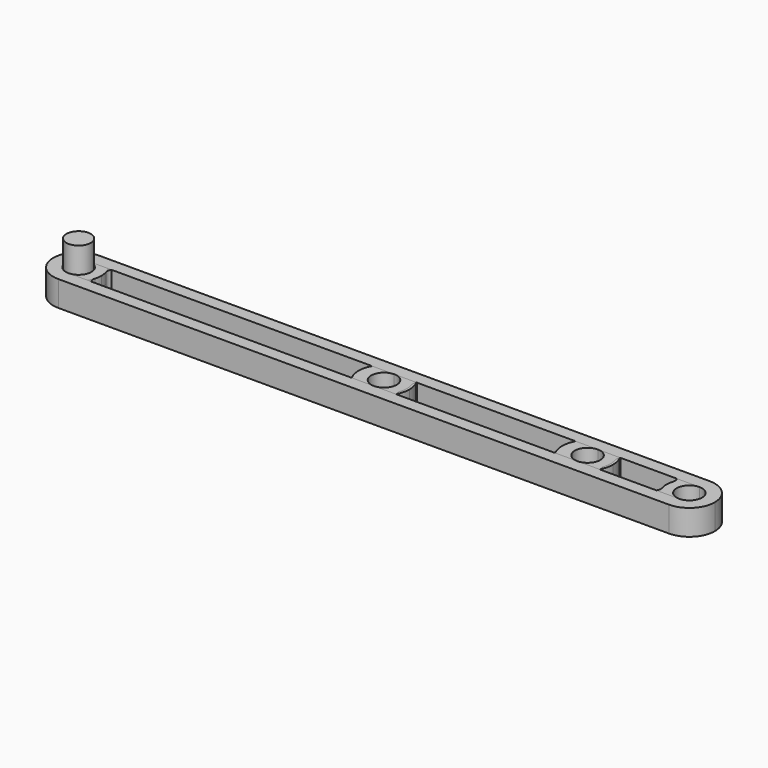
from build123d import *

# Parameters (mm, degrees)
F1_DEPTH      = 6.35
F2_DEPTH      = 6.35
F3_DEPTH      = 6.35
F4_DEPTH      = 6.35
F0_R          = 3.048
F5_DEPTH      = 12.7
F6_T          = -2.54
F7_T          = -2.54
F8_T          = -2.54
F9_T1_DEPTH   = 6.35
F9_2_T1_DEPTH = 6.35
F9_3_T1_DEPTH = 6.35


# Not quite as in the source:
# - a fillet or chamfer that OpenCascade refuses, or shapes differently, is made with other operations: its cross-section is extruded or revolved along the edge and cut away or added
# - two fillets or chamfers of one size are made in one step


with BuildPart() as f1:
    # F0 (on Top) → F1 (new body)
    with BuildSketch(Plane.XY):
        with BuildLine():
            ThreePointArc((0, 6.35), (3.175, 5.499261314), (5.499261314, 3.175))
            Line((5.499261314, 3.175), (70.700738686, 3.175))
            ThreePointArc((70.700738686, 3.175), (73.025, 5.499261314), (76.2, 6.35))
            Line((76.2, 6.35), (0, 6.35))
        make_face()
        with BuildLine():
            Line((76.2, 3.175), (70.700738686, 3.175))
            ThreePointArc((70.700738686, 3.175), (69.85, 0), (70.700738686, -3.175))
            Line((70.700738686, -3.175), (76.2, -3.175))
            ThreePointArc((76.2, -3.175), (73.025, 0), (76.2, 3.175))
        make_face()
        with BuildLine():
            Line((81.699261314, 3.175), (76.2, 3.175))
            ThreePointArc((76.2, 3.175), (78.4450640303, 2.2450640303), (79.375, 0))
            ThreePointArc((79.375, 0), (78.4450640303, -2.2450640303), (76.2, -3.175))
            Line((76.2, -3.175), (81.699261314, -3.175))
            ThreePointArc((81.699261314, -3.175), (82.3336289969, -1.6435009364), (82.55, 0))
            ThreePointArc((82.55, 0), (82.3336289969, 1.6435009364), (81.699261314, 3.175))
        make_face()
        with BuildLine():
            ThreePointArc((0, -3.175), (-3.175, 0), (0, 3.175))
            Line((0, 3.175), (5.499261314, 3.175))
            ThreePointArc((5.499261314, 3.175), (3.175, 5.499261314), (0, 6.35))
            ThreePointArc((0, 6.35), (-6.35, 0), (0, -6.35))
            ThreePointArc((0, -6.35), (3.175, -5.499261314), (5.499261314, -3.175))
            Line((5.499261314, -3.175), (0, -3.175))
        make_face()
        with BuildLine():
            ThreePointArc((0, 3.175), (2.2450640303, 2.2450640303), (3.175, 0))
            ThreePointArc((3.175, 0), (2.2450640303, -2.2450640303), (0, -3.175))
            Line((0, -3.175), (5.499261314, -3.175))
            ThreePointArc((5.499261314, -3.175), (6.1336289969, -1.6435009364), (6.35, 0))
            ThreePointArc((6.35, 0), (6.1336289969, 1.6435009364), (5.499261314, 3.175))
            Line((5.499261314, 3.175), (0, 3.175))
        make_face()
        with BuildLine():
            Line((70.700738686, 3.175), (5.499261314, 3.175))
            ThreePointArc((5.499261314, 3.175), (6.1336289969, 1.6435009364), (6.35, 0))
            ThreePointArc((6.35, 0), (6.1336289969, -1.6435009364), (5.499261314, -3.175))
            Line((5.499261314, -3.175), (70.700738686, -3.175))
            ThreePointArc((70.700738686, -3.175), (69.85, 0), (70.700738686, 3.175))
        make_face()
        with BuildLine():
            Line((70.700738686, -3.175), (5.499261314, -3.175))
            ThreePointArc((5.499261314, -3.175), (3.175, -5.499261314), (0, -6.35))
            Line((0, -6.35), (76.2, -6.35))
            ThreePointArc((76.2, -6.35), (73.025, -5.499261314), (70.700738686, -3.175))
        make_face()
        with BuildLine():
            ThreePointArc((76.2, 6.35), (73.025, 5.499261314), (70.700738686, 3.175))
            Line((70.700738686, 3.175), (76.2, 3.175))
            Line((76.2, 3.175), (81.699261314, 3.175))
            ThreePointArc((81.699261314, 3.175), (79.375, 5.499261314), (76.2, 6.35))
        make_face()
        with BuildLine():
            Line((76.2, -3.175), (70.700738686, -3.175))
            ThreePointArc((70.700738686, -3.175), (73.025, -5.499261314), (76.2, -6.35))
            ThreePointArc((76.2, -6.35), (79.375, -5.499261314), (81.699261314, -3.175))
            Line((81.699261314, -3.175), (76.2, -3.175))
        make_face()
    extrude(amount=F1_DEPTH)

    # F6: a shell. OpenCascade refuses it in one call, so the cavity is built on its own and cut out:
    # the body offset inwards by the wall thickness, plus a prism from it out through each open face.
    f6_core = offset(f1.part, amount=F6_T, mode=Mode.PRIVATE)
    f6_exits = [f6_core.faces().sort_by_distance(p)[0] for p in [
        (38.1, 0, 3.81),
        (38.1, 0, 2.54),
    ]]
    add(f6_core, mode=Mode.SUBTRACT)
    extrude(f6_exits, amount=-F6_T, mode=Mode.SUBTRACT)

    # F9: fillet of radius 1.5875 on 4 edges, made by hand

    # F9_s2 → F9_t1 (join)
    with BuildSketch(Plane.XY):
        with BuildLine():
            ThreePointArc((5.4438859411, -1.7393478261), (5.674054576, -3.1587564216), (6.9560764803, -3.81))
            Line((6.9560764803, -3.81), (4.2597094971, -3.81))
            ThreePointArc((4.2597094971, -3.81), (4.961032273, -2.8371435964), (5.4438859411, -1.7393478261))
        make_face()
        with BuildLine():
            ThreePointArc((5.4438859411, 1.7393478261), (5.674054576, 3.1587564216), (6.9560764803, 3.81))
            Line((6.9560764803, 3.81), (4.2597094971, 3.81))
            ThreePointArc((4.2597094971, 3.81), (4.961032273, 2.8371435964), (5.4438859411, 1.7393478261))
        make_face()
        with BuildLine():
            ThreePointArc((69.2439235197, 3.81), (70.525945424, 3.1587564216), (70.7561140589, 1.7393478261))
            ThreePointArc((70.7561140589, 1.7393478261), (71.238967727, 2.8371435964), (71.9402905029, 3.81))
            Line((71.9402905029, 3.81), (69.2439235197, 3.81))
        make_face()
        with BuildLine():
            ThreePointArc((70.7561140589, -1.7393478261), (70.525945424, -3.1587564216), (69.2439235197, -3.81))
            Line((69.2439235197, -3.81), (71.9402905029, -3.81))
            ThreePointArc((71.9402905029, -3.81), (71.238967727, -2.8371435964), (70.7561140589, -1.7393478261))
        make_face()
    extrude(amount=F9_T1_DEPTH)


with BuildPart() as f2:
    # F0 (on Top) → F2 (new body)
    with BuildSketch(Plane.XY):
        with BuildLine():
            Line((127, 6.35), (76.2, 6.35))
            ThreePointArc((76.2, 6.35), (79.375, 5.499261314), (81.699261314, 3.175))
            Line((81.699261314, 3.175), (121.500738686, 3.175))
            ThreePointArc((121.500738686, 3.175), (123.825, 5.499261314), (127, 6.35))
        make_face()
        with BuildLine():
            Line((121.500738686, 3.175), (81.699261314, 3.175))
            ThreePointArc((81.699261314, 3.175), (82.3336289969, 1.6435009364), (82.55, 0))
            ThreePointArc((82.55, 0), (82.3336289969, -1.6435009364), (81.699261314, -3.175))
            Line((81.699261314, -3.175), (121.500738686, -3.175))
            ThreePointArc((121.500738686, -3.175), (120.65, 0), (121.500738686, 3.175))
        make_face()
        with BuildLine():
            ThreePointArc((81.699261314, -3.175), (79.375, -5.499261314), (76.2, -6.35))
            Line((76.2, -6.35), (127, -6.35))
            ThreePointArc((127, -6.35), (123.825, -5.499261314), (121.500738686, -3.175))
            Line((121.500738686, -3.175), (81.699261314, -3.175))
        make_face()
        with BuildLine():
            Line((127, 3.175), (121.500738686, 3.175))
            ThreePointArc((121.500738686, 3.175), (120.65, 0), (121.500738686, -3.175))
            Line((121.500738686, -3.175), (127, -3.175))
            ThreePointArc((127, -3.175), (123.825, 0), (127, 3.175))
        make_face()
        with BuildLine():
            ThreePointArc((132.499261314, 3.175), (130.175, 5.499261314), (127, 6.35))
            ThreePointArc((127, 6.35), (123.825, 5.499261314), (121.500738686, 3.175))
            Line((121.500738686, 3.175), (127, 3.175))
            Line((127, 3.175), (132.499261314, 3.175))
        make_face()
        with BuildLine():
            ThreePointArc((133.35, 0), (133.1336289969, 1.6435009364), (132.499261314, 3.175))
            Line((132.499261314, 3.175), (127, 3.175))
            ThreePointArc((127, 3.175), (129.2450640303, 2.2450640303), (130.175, 0))
            ThreePointArc((130.175, 0), (129.2450640303, -2.2450640303), (127, -3.175))
            Line((127, -3.175), (132.499261314, -3.175))
            ThreePointArc((132.499261314, -3.175), (133.1336289969, -1.6435009364), (133.35, 0))
        make_face()
        with BuildLine():
            ThreePointArc((121.500738686, -3.175), (123.825, -5.499261314), (127, -6.35))
            ThreePointArc((127, -6.35), (130.175, -5.499261314), (132.499261314, -3.175))
            Line((132.499261314, -3.175), (127, -3.175))
            Line((127, -3.175), (121.500738686, -3.175))
        make_face()
        with BuildLine():
            ThreePointArc((76.2, 6.35), (73.025, 5.499261314), (70.700738686, 3.175))
            Line((70.700738686, 3.175), (76.2, 3.175))
            Line((76.2, 3.175), (81.699261314, 3.175))
            ThreePointArc((81.699261314, 3.175), (79.375, 5.499261314), (76.2, 6.35))
        make_face()
        with BuildLine():
            Line((76.2, 3.175), (70.700738686, 3.175))
            ThreePointArc((70.700738686, 3.175), (69.85, 0), (70.700738686, -3.175))
            Line((70.700738686, -3.175), (76.2, -3.175))
            ThreePointArc((76.2, -3.175), (73.025, 0), (76.2, 3.175))
        make_face()
        with BuildLine():
            Line((81.699261314, 3.175), (76.2, 3.175))
            ThreePointArc((76.2, 3.175), (78.4450640303, 2.2450640303), (79.375, 0))
            ThreePointArc((79.375, 0), (78.4450640303, -2.2450640303), (76.2, -3.175))
            Line((76.2, -3.175), (81.699261314, -3.175))
            ThreePointArc((81.699261314, -3.175), (82.3336289969, -1.6435009364), (82.55, 0))
            ThreePointArc((82.55, 0), (82.3336289969, 1.6435009364), (81.699261314, 3.175))
        make_face()
        with BuildLine():
            Line((76.2, -3.175), (70.700738686, -3.175))
            ThreePointArc((70.700738686, -3.175), (73.025, -5.499261314), (76.2, -6.35))
            ThreePointArc((76.2, -6.35), (79.375, -5.499261314), (81.699261314, -3.175))
            Line((81.699261314, -3.175), (76.2, -3.175))
        make_face()
    extrude(amount=F2_DEPTH)

    # F7: a shell. OpenCascade refuses it in one call, so the cavity is built on its own and cut out:
    # the body offset inwards by the wall thickness, plus a prism from it out through each open face.
    f7_core = offset(f2.part, amount=F7_T, mode=Mode.PRIVATE)
    f7_exits = [f7_core.faces().sort_by_distance(p)[0] for p in [
        (101.6, 0, 3.81),
        (101.6, 0, 2.54),
    ]]
    add(f7_core, mode=Mode.SUBTRACT)
    extrude(f7_exits, amount=-F7_T, mode=Mode.SUBTRACT)

    # F9#2: fillet of radius 1.5875 on 4 edges, made by hand

    # F9_2_s2 → F9_2_t1 (join)
    with BuildSketch(Plane.XY):
        with BuildLine():
            ThreePointArc((120.0439235197, -3.81), (121.325945424, -3.1587564216), (121.5561140589, -1.7393478261))
            ThreePointArc((121.5561140589, -1.7393478261), (122.038967727, -2.8371435964), (122.7402905029, -3.81))
            Line((122.7402905029, -3.81), (120.0439235197, -3.81))
        make_face()
        with BuildLine():
            ThreePointArc((83.1560764803, -3.81), (81.874054576, -3.1587564216), (81.6438859411, -1.7393478261))
            ThreePointArc((81.6438859411, -1.7393478261), (81.161032273, -2.8371435964), (80.4597094971, -3.81))
            Line((80.4597094971, -3.81), (83.1560764803, -3.81))
        make_face()
        with BuildLine():
            ThreePointArc((81.6438859411, 1.7393478261), (81.874054576, 3.1587564216), (83.1560764803, 3.81))
            Line((83.1560764803, 3.81), (80.4597094971, 3.81))
            ThreePointArc((80.4597094971, 3.81), (81.161032273, 2.8371435964), (81.6438859411, 1.7393478261))
        make_face()
        with BuildLine():
            ThreePointArc((120.0439235197, 3.81), (121.325945424, 3.1587564216), (121.5561140589, 1.7393478261))
            ThreePointArc((121.5561140589, 1.7393478261), (122.038967727, 2.8371435964), (122.7402905029, 3.81))
            Line((122.7402905029, 3.81), (120.0439235197, 3.81))
        make_face()
    extrude(amount=F9_2_T1_DEPTH)


with BuildPart() as f3:
    # F0 (on Top) → F3 (new body)
    with BuildSketch(Plane.XY):
        with BuildLine():
            Line((152.4, 6.35), (127, 6.35))
            ThreePointArc((127, 6.35), (130.175, 5.499261314), (132.499261314, 3.175))
            Line((132.499261314, 3.175), (146.900738686, 3.175))
            ThreePointArc((146.900738686, 3.175), (149.225, 5.499261314), (152.4, 6.35))
        make_face()
        with BuildLine():
            Line((127, 3.175), (121.500738686, 3.175))
            ThreePointArc((121.500738686, 3.175), (120.65, 0), (121.500738686, -3.175))
            Line((121.500738686, -3.175), (127, -3.175))
            ThreePointArc((127, -3.175), (123.825, 0), (127, 3.175))
        make_face()
        with BuildLine():
            ThreePointArc((133.35, 0), (133.1336289969, 1.6435009364), (132.499261314, 3.175))
            Line((132.499261314, 3.175), (127, 3.175))
            ThreePointArc((127, 3.175), (129.2450640303, 2.2450640303), (130.175, 0))
            ThreePointArc((130.175, 0), (129.2450640303, -2.2450640303), (127, -3.175))
            Line((127, -3.175), (132.499261314, -3.175))
            ThreePointArc((132.499261314, -3.175), (133.1336289969, -1.6435009364), (133.35, 0))
        make_face()
        with BuildLine():
            Line((152.4, 3.175), (146.900738686, 3.175))
            ThreePointArc((146.900738686, 3.175), (146.05, 0), (146.900738686, -3.175))
            Line((146.900738686, -3.175), (152.4, -3.175))
            ThreePointArc((152.4, -3.175), (149.225, 0), (152.4, 3.175))
        make_face()
        with BuildLine():
            ThreePointArc((158.75, 0), (156.8901280605, 4.4901280605), (152.4, 6.35))
            ThreePointArc((152.4, 6.35), (149.225, 5.499261314), (146.900738686, 3.175))
            Line((146.900738686, 3.175), (152.4, 3.175))
            ThreePointArc((152.4, 3.175), (154.6450640303, 2.2450640303), (155.575, 0))
            ThreePointArc((155.575, 0), (154.6450640303, -2.2450640303), (152.4, -3.175))
            Line((152.4, -3.175), (146.900738686, -3.175))
            ThreePointArc((146.900738686, -3.175), (149.225, -5.499261314), (152.4, -6.35))
            ThreePointArc((152.4, -6.35), (156.8901280605, -4.4901280605), (158.75, 0))
        make_face()
        with BuildLine():
            Line((146.900738686, 3.175), (132.499261314, 3.175))
            ThreePointArc((132.499261314, 3.175), (133.1336289969, 1.6435009364), (133.35, 0))
            ThreePointArc((133.35, 0), (133.1336289969, -1.6435009364), (132.499261314, -3.175))
            Line((132.499261314, -3.175), (146.900738686, -3.175))
            ThreePointArc((146.900738686, -3.175), (146.05, 0), (146.900738686, 3.175))
        make_face()
        with BuildLine():
            ThreePointArc((132.499261314, -3.175), (130.175, -5.499261314), (127, -6.35))
            Line((127, -6.35), (152.4, -6.35))
            ThreePointArc((152.4, -6.35), (149.225, -5.499261314), (146.900738686, -3.175))
            Line((146.900738686, -3.175), (132.499261314, -3.175))
        make_face()
        with BuildLine():
            ThreePointArc((132.499261314, 3.175), (130.175, 5.499261314), (127, 6.35))
            ThreePointArc((127, 6.35), (123.825, 5.499261314), (121.500738686, 3.175))
            Line((121.500738686, 3.175), (127, 3.175))
            Line((127, 3.175), (132.499261314, 3.175))
        make_face()
        with BuildLine():
            ThreePointArc((121.500738686, -3.175), (123.825, -5.499261314), (127, -6.35))
            ThreePointArc((127, -6.35), (130.175, -5.499261314), (132.499261314, -3.175))
            Line((132.499261314, -3.175), (127, -3.175))
            Line((127, -3.175), (121.500738686, -3.175))
        make_face()
    extrude(amount=F3_DEPTH)

    # F8: a shell. OpenCascade refuses it in one call, so the cavity is built on its own and cut out:
    # the body offset inwards by the wall thickness, plus a prism from it out through each open face.
    f8_core = offset(f3.part, amount=F8_T, mode=Mode.PRIVATE)
    f8_exits = [f8_core.faces().sort_by_distance(p)[0] for p in [
        (139.7, 0, 3.81),
        (139.7, 0, 2.54),
    ]]
    add(f8_core, mode=Mode.SUBTRACT)
    extrude(f8_exits, amount=-F8_T, mode=Mode.SUBTRACT)

    # F9#3: fillet of radius 1.5875 on 4 edges, made by hand

    # F9_3_s2 → F9_3_t1 (join)
    with BuildSketch(Plane.XY):
        with BuildLine():
            ThreePointArc((133.9560764803, -3.81), (132.674054576, -3.1587564216), (132.4438859411, -1.7393478261))
            ThreePointArc((132.4438859411, -1.7393478261), (131.961032273, -2.8371435964), (131.2597094971, -3.81))
            Line((131.2597094971, -3.81), (133.9560764803, -3.81))
        make_face()
        with BuildLine():
            ThreePointArc((145.4439235197, -3.81), (146.725945424, -3.1587564216), (146.9561140589, -1.7393478261))
            ThreePointArc((146.9561140589, -1.7393478261), (147.438967727, -2.8371435964), (148.1402905029, -3.81))
            Line((148.1402905029, -3.81), (145.4439235197, -3.81))
        make_face()
        with BuildLine():
            ThreePointArc((132.4438859411, 1.7393478261), (132.674054576, 3.1587564216), (133.9560764803, 3.81))
            Line((133.9560764803, 3.81), (131.2597094971, 3.81))
            ThreePointArc((131.2597094971, 3.81), (131.961032273, 2.8371435964), (132.4438859411, 1.7393478261))
        make_face()
        with BuildLine():
            ThreePointArc((145.4439235197, 3.81), (146.725945424, 3.1587564216), (146.9561140589, 1.7393478261))
            ThreePointArc((146.9561140589, 1.7393478261), (147.438967727, 2.8371435964), (148.1402905029, 3.81))
            Line((148.1402905029, 3.81), (145.4439235197, 3.81))
        make_face()
    extrude(amount=F9_3_T1_DEPTH)


with BuildPart() as f4:
    # F0 (on Top) → F4 (new body)
    with BuildSketch(Plane.XY):
        with BuildLine():
            ThreePointArc((0, -3.175), (-3.175, 0), (0, 3.175))
            Line((0, 3.175), (5.499261314, 3.175))
            ThreePointArc((5.499261314, 3.175), (3.175, 5.499261314), (0, 6.35))
            ThreePointArc((0, 6.35), (-6.35, 0), (0, -6.35))
            ThreePointArc((0, -6.35), (3.175, -5.499261314), (5.499261314, -3.175))
            Line((5.499261314, -3.175), (0, -3.175))
        make_face()
        with BuildLine():
            ThreePointArc((0, 6.35), (3.175, 5.499261314), (5.499261314, 3.175))
            Line((5.499261314, 3.175), (70.700738686, 3.175))
            ThreePointArc((70.700738686, 3.175), (73.025, 5.499261314), (76.2, 6.35))
            Line((76.2, 6.35), (0, 6.35))
        make_face()
        with BuildLine():
            ThreePointArc((76.2, 6.35), (73.025, 5.499261314), (70.700738686, 3.175))
            Line((70.700738686, 3.175), (76.2, 3.175))
            Line((76.2, 3.175), (81.699261314, 3.175))
            ThreePointArc((81.699261314, 3.175), (79.375, 5.499261314), (76.2, 6.35))
        make_face()
        with BuildLine():
            Line((70.700738686, -3.175), (5.499261314, -3.175))
            ThreePointArc((5.499261314, -3.175), (3.175, -5.499261314), (0, -6.35))
            Line((0, -6.35), (76.2, -6.35))
            ThreePointArc((76.2, -6.35), (73.025, -5.499261314), (70.700738686, -3.175))
        make_face()
        with BuildLine():
            Line((76.2, -3.175), (70.700738686, -3.175))
            ThreePointArc((70.700738686, -3.175), (73.025, -5.499261314), (76.2, -6.35))
            ThreePointArc((76.2, -6.35), (79.375, -5.499261314), (81.699261314, -3.175))
            Line((81.699261314, -3.175), (76.2, -3.175))
        make_face()
        with BuildLine():
            Line((127, 6.35), (76.2, 6.35))
            ThreePointArc((76.2, 6.35), (79.375, 5.499261314), (81.699261314, 3.175))
            Line((81.699261314, 3.175), (121.500738686, 3.175))
            ThreePointArc((121.500738686, 3.175), (123.825, 5.499261314), (127, 6.35))
        make_face()
        with BuildLine():
            ThreePointArc((132.499261314, 3.175), (130.175, 5.499261314), (127, 6.35))
            ThreePointArc((127, 6.35), (123.825, 5.499261314), (121.500738686, 3.175))
            Line((121.500738686, 3.175), (127, 3.175))
            Line((127, 3.175), (132.499261314, 3.175))
        make_face()
        with BuildLine():
            Line((152.4, 6.35), (127, 6.35))
            ThreePointArc((127, 6.35), (130.175, 5.499261314), (132.499261314, 3.175))
            Line((132.499261314, 3.175), (146.900738686, 3.175))
            ThreePointArc((146.900738686, 3.175), (149.225, 5.499261314), (152.4, 6.35))
        make_face()
        with BuildLine():
            ThreePointArc((158.75, 0), (156.8901280605, 4.4901280605), (152.4, 6.35))
            ThreePointArc((152.4, 6.35), (149.225, 5.499261314), (146.900738686, 3.175))
            Line((146.900738686, 3.175), (152.4, 3.175))
            ThreePointArc((152.4, 3.175), (154.6450640303, 2.2450640303), (155.575, 0))
            ThreePointArc((155.575, 0), (154.6450640303, -2.2450640303), (152.4, -3.175))
            Line((152.4, -3.175), (146.900738686, -3.175))
            ThreePointArc((146.900738686, -3.175), (149.225, -5.499261314), (152.4, -6.35))
            ThreePointArc((152.4, -6.35), (156.8901280605, -4.4901280605), (158.75, 0))
        make_face()
        with BuildLine():
            ThreePointArc((132.499261314, -3.175), (130.175, -5.499261314), (127, -6.35))
            Line((127, -6.35), (152.4, -6.35))
            ThreePointArc((152.4, -6.35), (149.225, -5.499261314), (146.900738686, -3.175))
            Line((146.900738686, -3.175), (132.499261314, -3.175))
        make_face()
        with BuildLine():
            ThreePointArc((121.500738686, -3.175), (123.825, -5.499261314), (127, -6.35))
            ThreePointArc((127, -6.35), (130.175, -5.499261314), (132.499261314, -3.175))
            Line((132.499261314, -3.175), (127, -3.175))
            Line((127, -3.175), (121.500738686, -3.175))
        make_face()
        with BuildLine():
            ThreePointArc((81.699261314, -3.175), (79.375, -5.499261314), (76.2, -6.35))
            Line((76.2, -6.35), (127, -6.35))
            ThreePointArc((127, -6.35), (123.825, -5.499261314), (121.500738686, -3.175))
            Line((121.500738686, -3.175), (81.699261314, -3.175))
        make_face()
    extrude(amount=F4_DEPTH)


with BuildPart() as f5:
    # F0 (on Top) → F5 (new body)
    with BuildSketch(Plane.XY):
        Circle(F0_R)
    extrude(amount=F5_DEPTH)


solid = Compound([f1.part, f2.part, f3.part, f4.part, f5.part])
